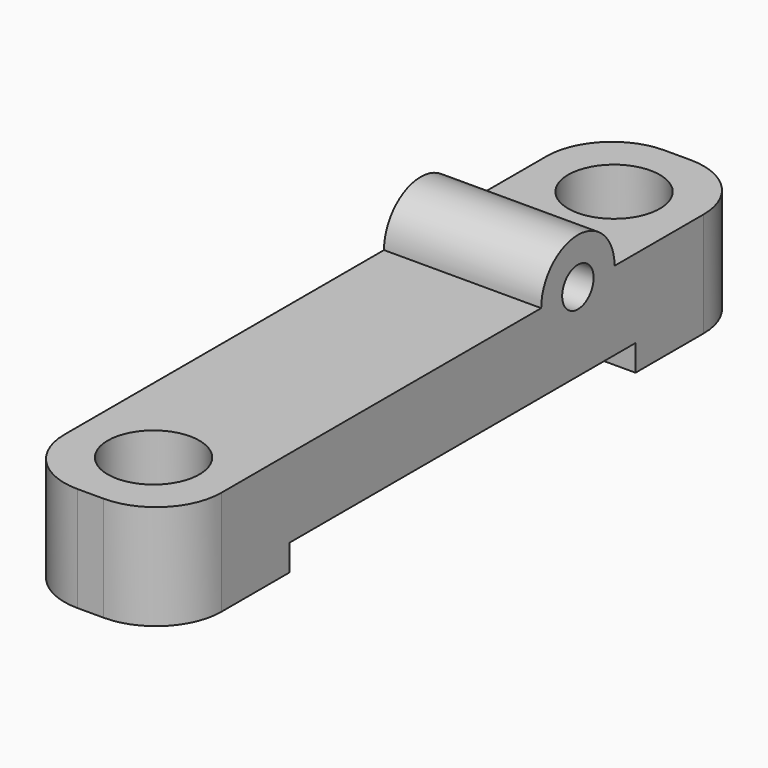
from build123d import *

# Parameters (mm, degrees)
F0_W     = 1.25
F0_H     = 4
F0_W_2   = 1.75
F1_DEPTH = 6
F4_DEPTH = 4
F5_DEPTH = 4
F6_DEPTH = 4


# Not quite as in the source:
# - a feature names something its author has since deleted; it is built from what else it names


with BuildPart() as f1:
    # F0 (on Right) → F1 (new body)
    with BuildSketch(Plane.YZ):
        with Locations((-34.0711950026, -0.2365471814)):
            Rectangle(F0_W, F0_H)
        with Locations((-35.5711950026, -0.2365471814)):
            Rectangle(F0_W_2, F0_H)
        with BuildLine():
            Line((-38.1961950026, -2.2365471814), (-36.4461950026, -2.2365471814))
            Line((-36.4461950026, -2.2365471814), (-36.4461950026, 1.7634528186))
            Line((-36.4461950026, 1.7634528186), (-38.1961950026, 1.7634528186))
            Line((-38.1961950026, 1.7634528186), (-40.1961950026, 1.7634528186))
            ThreePointArc((-40.1961950026, 1.7634528186), (-41.9461950026, 0.0134528186), (-43.6961950026, 1.7634528186))
            Line((-43.6961950026, 1.7634528186), (-56.6961950026, 1.7634528186))
            Line((-56.6961950026, 1.7634528186), (-56.6961950026, -1.4865471814))
            Line((-56.6961950026, -1.4865471814), (-56.6961950026, -2.2365471814))
            Line((-56.6961950026, -2.2365471814), (-55.6961950026, -2.2365471814))
            Line((-55.6961950026, -2.2365471814), (-55.6961950026, -1.2365471814))
            Line((-55.6961950026, -1.2365471814), (-39.1961950026, -1.2365471814))
            Line((-39.1961950026, -1.2365471814), (-39.1961950026, -2.2365471814))
            Line((-39.1961950026, -2.2365471814), (-38.1961950026, -2.2365471814))
        make_face()
        with BuildLine():
            ThreePointArc((-43.6961950026, 1.7634528186), (-41.9461950026, 0.0134528186), (-40.1961950026, 1.7634528186))
            Line((-40.1961950026, 1.7634528186), (-41.1961950026, 1.7634528186))
            ThreePointArc((-41.1961950026, 1.7634528186), (-41.9461950026, 1.0134528186), (-42.6961950026, 1.7634528186))
            Line((-42.6961950026, 1.7634528186), (-43.6961950026, 1.7634528186))
        make_face()
        with BuildLine():
            Line((-41.1961950026, 1.7634528186), (-40.1961950026, 1.7634528186))
            ThreePointArc((-40.1961950026, 1.7634528186), (-41.9461950026, 3.5134528186), (-43.6961950026, 1.7634528186))
            Line((-43.6961950026, 1.7634528186), (-42.6961950026, 1.7634528186))
            ThreePointArc((-42.6961950026, 1.7634528186), (-41.9461950026, 2.5134528186), (-41.1961950026, 1.7634528186))
        make_face()
        Polygon((-56.6961950026, -1.4865471814), (-56.6961950026, 1.7634528186), (-58.4461950026, 1.7634528186), (-58.4461950026, -2.2365471814), (-56.6961950026, -2.2365471814), align=None)
        with Locations((-59.3211950026, -0.2365471814)):
            Rectangle(F0_W_2, F0_H)
        Polygon((-60.1961950026, -2.2365471814), (-60.1961950026, 1.7634528186), (-61.4461950026, 1.7634528186), (-61.4461950026, -0.2365471814), (-61.4461950026, -2.2365471814), align=None)
    extrude(amount=F1_DEPTH)

    # F2 (on face) → F4 (cut)
    with BuildSketch(Plane(origin=(0, 0, -2.2365471814), x_dir=(1, 0, 0), z_dir=(0, 0, -1))):
        with BuildLine():
            Line((0, 61.4461950026), (0, 58.9461950026))
            ThreePointArc((0, 58.9461950026), (0.732233047, 60.7139619556), (2.5, 61.4461950026))
            Line((2.5, 61.4461950026), (0, 61.4461950026))
        make_face()
        with BuildLine():
            ThreePointArc((3.5, 61.4461950026), (5.267766953, 60.7139619556), (6, 58.9461950026))
            Line((6, 58.9461950026), (6, 61.4461950026))
            Line((6, 61.4461950026), (3.5, 61.4461950026))
        make_face()
    extrude(amount=-F4_DEPTH, mode=Mode.SUBTRACT)

    # F2 (on face) → F5 (cut)
    with BuildSketch(Plane(origin=(0, 0, -2.2365471814), x_dir=(1, 0, 0), z_dir=(0, 0, -1))):
        with BuildLine():
            Line((1.25, 58.4407150745), (4.75, 58.4407150745))
            ThreePointArc((4.75, 58.4407150745), (3, 60.1907150745), (1.25, 58.4407150745))
        make_face()
        with BuildLine():
            ThreePointArc((1.25, 58.4407150745), (3, 56.6907150745), (4.75, 58.4407150745))
            Line((4.75, 58.4407150745), (1.25, 58.4407150745))
        make_face()
    extrude(amount=-F5_DEPTH, mode=Mode.SUBTRACT)

    # F3 (on face) → F6 (cut)
    with BuildSketch(Plane(origin=(0, 0, -2.2365471814), x_dir=(1, 0, 0), z_dir=(0, 0, -1))):
        with BuildLine():
            Line((1.25, 36.4720486104), (4.75, 36.4720486104))
            ThreePointArc((4.75, 36.4720486104), (3, 38.2220486104), (1.25, 36.4720486104))
        make_face()
        with BuildLine():
            Line((6, 33.4461950026), (6, 35.9461950026))
            ThreePointArc((6, 35.9461950026), (5.267766953, 34.1784280497), (3.5, 33.4461950026))
            Line((3.5, 33.4461950026), (6, 33.4461950026))
        make_face()
        with BuildLine():
            ThreePointArc((2.5, 33.4461950026), (0.732233047, 34.1784280497), (0, 35.9461950026))
            Line((0, 35.9461950026), (0, 33.4461950026))
            Line((0, 33.4461950026), (2.5, 33.4461950026))
        make_face()
        with BuildLine():
            ThreePointArc((1.25, 36.4720486104), (3, 34.7220486104), (4.75, 36.4720486104))
            Line((4.75, 36.4720486104), (1.25, 36.4720486104))
        make_face()
    extrude(amount=-F6_DEPTH, mode=Mode.SUBTRACT)


solid = f1.part
